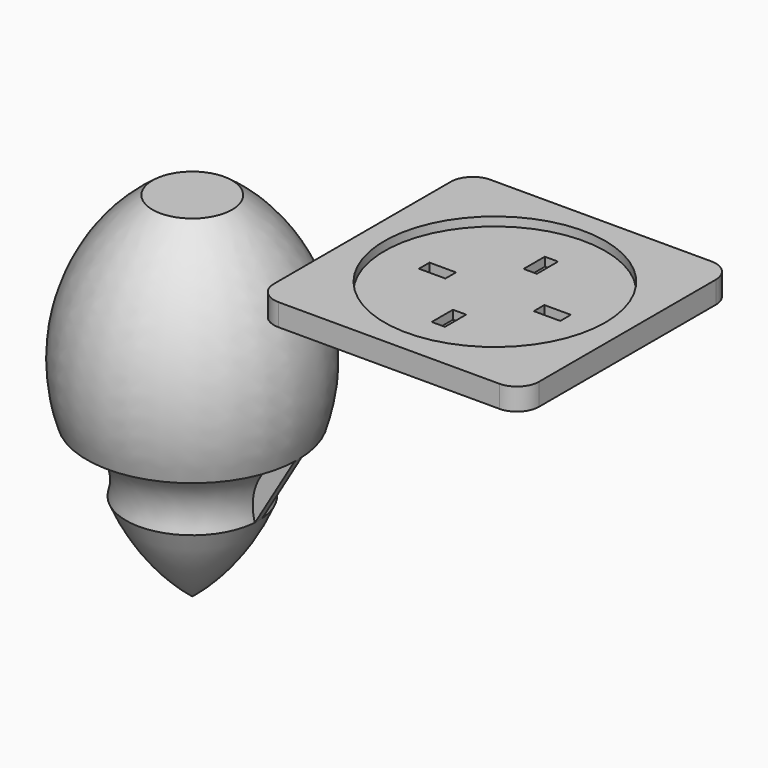
from build123d import *

# Parameters (mm, degrees)
F0_W      = 60
F0_H      = 60
F1_DEPTH  = 5
F2_R      = 25
F3_DEPTH  = 2
F4_R      = 5
F5_W      = 6
F5_H      = 3
F5_W_2    = 3
F5_H_2    = 6
F6_DEPTH  = 2
F7_W      = 7
F7_H      = 2
F10_DEPTH = 1


# Not quite as in the source:
# - a feature names something its author has since deleted; it is built from what else it names


with BuildPart() as f1:
    # F0 (on Top) → F1 (new body)
    with BuildSketch(Plane.XY):
        Rectangle(F0_W, F0_H)
    extrude(amount=F1_DEPTH)

    # F2 (on face) → F3 (cut)
    with BuildSketch(Plane.XY.offset(5)):
        Circle(F2_R)
    extrude(amount=-F3_DEPTH, mode=Mode.SUBTRACT)

    # F4
    f4_edges = [f1.edges().sort_by_distance(p)[0] for p in [
        (-30, -30, 2.5),
        (30, -30, 2.5),
        (30, 30, 2.5),
        (-30, 30, 2.5),
    ]]
    fillet(f4_edges, radius=F4_R)

    # F5 (on face) → F6 (cut)
    with BuildSketch(Plane.XY.offset(3)):
        with Locations((-13, 0)):
            Rectangle(F5_W, F5_H)
        with Locations((0, 13)):
            Rectangle(F5_W_2, F5_H_2)
        with Locations((13, 0)):
            Rectangle(F5_W, F5_H)
        with Locations((0, -13)):
            Rectangle(F5_W_2, F5_H_2)
    extrude(amount=-F6_DEPTH, mode=Mode.SUBTRACT)


with BuildPart() as f8:
    # F7 (on Front) → F8 (revolve)
    with BuildSketch(Plane.XZ):
        with Locations((-65.0005573104, -1)):
            Rectangle(F7_W, F7_H)
        with BuildLine():
            Line((-61.5005573104, -2), (-68.5005573104, -2))
            Line((-68.5005573104, -2), (-68.5005573104, -45))
            Line((-68.5005573104, -45), (-44.6224203376, -45))
            ThreePointArc((-44.6224203376, -45), (-44.6789062027, -20.0591316566), (-59.5005573104, 0))
            Line((-59.5005573104, 0), (-61.5005573104, 0))
            Line((-61.5005573104, 0), (-61.5005573104, -2))
        make_face()
        with BuildLine():
            Line((-44.6224203376, -45), (-68.5005573104, -45))
            Line((-68.5005573104, -45), (-68.5005573104, -60))
            Line((-68.5005573104, -60), (-53.5005573104, -60))
            ThreePointArc((-53.5005573104, -60), (-52.2895260676, -50.5894028799), (-44.6224203376, -45))
        make_face()
        with BuildLine():
            Line((-53.5005573104, -60), (-68.5005573104, -60))
            Line((-68.5005573104, -60), (-68.5005573104, -80))
            ThreePointArc((-68.5005573104, -80), (-59.7303907725, -70.9526249034), (-53.5005573104, -60))
        make_face()
    revolve(axis=Axis((-68.5005573104, 0, -40), (0, 0, -1)))


with BuildPart() as f10:
    # F9 (on Front) → F10 (new body, symmetric)
    with BuildSketch(Plane.XZ):
        Polygon((-44.6224203376, -45), (-92.3786942832, -45), (-83.5005573104, -60), (-53.5005573104, -60), align=None)
    extrude(amount=F10_DEPTH, both=True)


solid = Compound([f1.part, f8.part, f10.part])
